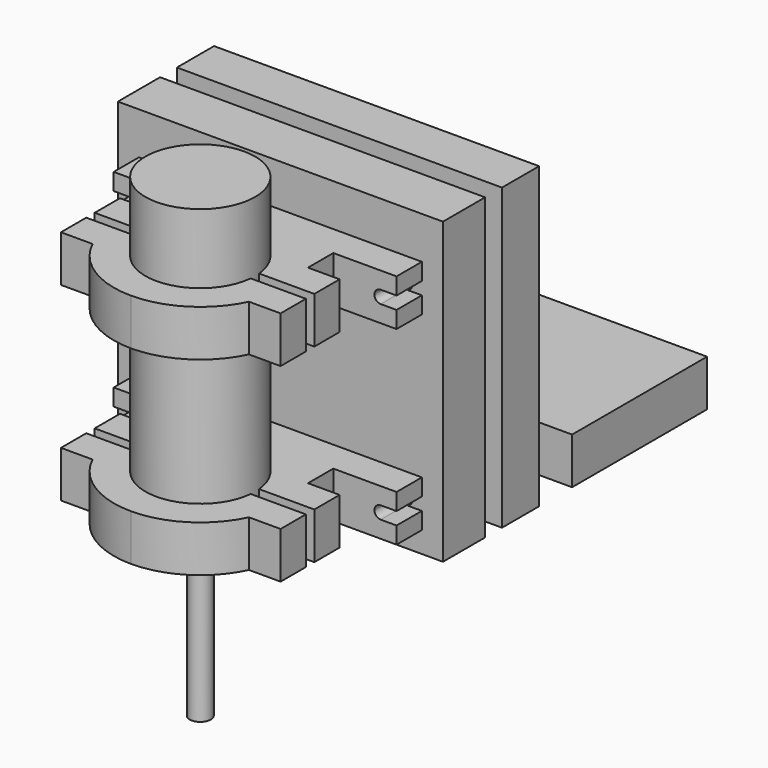
from build123d import *

# Parameters (mm, degrees)
F0_R      = 26
F0_R_2    = 5
F1_DEPTH  = 145
F2_DEPTH  = 80
F4_DEPTH  = 22
F6_DEPTH  = 88.501
F9_R      = 3
F10_DEPTH = 25
F12_W     = 154.1552425658
F12_H     = 142
F13_DEPTH = 22
F14_W     = 154.1552425658
F14_H     = 80
F15_DEPTH = 22


with BuildPart() as f1:
    # F0 (on Top) → F1 (new body)
    with BuildSketch(Plane.XY):
        Circle(F0_R)
        Circle(F0_R_2, mode=Mode.SUBTRACT)
        Circle(F0_R_2)
    extrude(amount=F1_DEPTH)

    # F0 (on Top) → F2 (join)
    with BuildSketch(Plane.XY):
        Circle(F0_R_2)
    extrude(amount=-F2_DEPTH)


with BuildPart() as f4:
    # F3 (on Top) → F4 (new body)
    with BuildSketch(Plane.XY):
        with BuildLine():
            ThreePointArc((25.8795285892, -2.5), (0, -26), (-25.8795285892, -2.5))
            Line((-25.8795285892, -2.5), (-52.0776212829, -2.5))
            Line((-52.0776212829, -2.5), (-52.0776212829, -17.5))
            Line((-52.0776212829, -17.5), (-37.0776212829, -17.5))
            ThreePointArc((-37.0776212829, -17.5), (-21.9488040676, -34.6301891418), (0, -41))
            ThreePointArc((0, -41), (21.9488040676, -34.6301891418), (37.0776212829, -17.5))
            Line((37.0776212829, -17.5), (52.0776212829, -17.5))
            Line((52.0776212829, -17.5), (52.0776212829, -2.5))
            Line((52.0776212829, -2.5), (25.8795285892, -2.5))
        make_face()
    extrude(amount=F4_DEPTH)


with BuildPart() as f4b:
    # F3 (on Top) → F4, piece 2 (new body)
    with BuildSketch(Plane.XY):
        with BuildLine():
            Line((-52.0776212829, 2.5), (-25.8795285892, 2.5))
            ThreePointArc((-25.8795285892, 2.5), (0, 26), (25.8795285892, 2.5))
            Line((25.8795285892, 2.5), (52.0776212829, 2.5))
            Line((52.0776212829, 2.5), (52.0776212829, 17.5))
            Line((52.0776212829, 17.5), (37.0776212829, 17.5))
            Line((37.0776212829, 17.5), (37.0776212829, 32.5))
            Line((37.0776212829, 32.5), (67.0776212829, 32.5))
            Line((67.0776212829, 32.5), (67.0776212829, 47.5))
            Line((67.0776212829, 47.5), (0, 47.5))
            Line((0, 47.5), (-67.0776212829, 47.5))
            Line((-67.0776212829, 47.5), (-67.0776212829, 32.5))
            Line((-67.0776212829, 32.5), (-37.0776212829, 32.5))
            Line((-37.0776212829, 32.5), (-37.0776212829, 17.5))
            Line((-37.0776212829, 17.5), (-52.0776212829, 17.5))
            Line((-52.0776212829, 17.5), (-52.0776212829, 2.5))
        make_face()
    extrude(amount=F4_DEPTH)

    # F5 (on face) → F6 (cut, through all)
    with BuildSketch(Plane(origin=(0, 47.5, 0), x_dir=(-1, 0, 0), z_dir=(0, 1, 0))):
        with BuildLine():
            ThreePointArc((-59.5776212829, 8), (-57.4563009394, 8.8786796564), (-56.5776212829, 11))
            ThreePointArc((-56.5776212829, 11), (-57.4563009394, 13.1213203436), (-59.5776212829, 14))
            ThreePointArc((-59.5776212829, 14), (-61.6989416265, 13.1213203436), (-62.5776212829, 11))
            ThreePointArc((-62.5776212829, 11), (-61.6989416265, 8.8786796564), (-59.5776212829, 8))
        make_face()
        with BuildLine():
            ThreePointArc((-62.5776212829, 11), (-61.6989416265, 13.1213203436), (-59.5776212829, 14))
            Line((-59.5776212829, 14), (-67.0776212829, 14))
            Line((-67.0776212829, 14), (-67.0776212829, 8))
            Line((-67.0776212829, 8), (-59.5776212829, 8))
            ThreePointArc((-59.5776212829, 8), (-61.6989416265, 8.8786796564), (-62.5776212829, 11))
        make_face()
        with BuildLine():
            ThreePointArc((59.5776212829, 14), (57.4563009394, 13.1213203436), (56.5776212829, 11))
            ThreePointArc((56.5776212829, 11), (57.4563009394, 8.8786796564), (59.5776212829, 8))
            ThreePointArc((59.5776212829, 8), (61.6989416265, 8.8786796564), (62.5776212829, 11))
            ThreePointArc((62.5776212829, 11), (61.6989416265, 13.1213203436), (59.5776212829, 14))
        make_face()
        with BuildLine():
            Line((67.0776212829, 14), (59.5776212829, 14))
            ThreePointArc((59.5776212829, 14), (61.6989416265, 13.1213203436), (62.5776212829, 11))
            ThreePointArc((62.5776212829, 11), (61.6989416265, 8.8786796564), (59.5776212829, 8))
            Line((59.5776212829, 8), (67.0776212829, 8))
            Line((67.0776212829, 8), (67.0776212829, 14))
        make_face()
    extrude(amount=-F6_DEPTH, mode=Mode.SUBTRACT)


with BuildPart() as f7_1:
    # F7: copy of F4
    add(f4.part.moved(Location((0, 0, 90))))


with BuildPart() as f8_1:
    # F8: copy of F4b
    add(f4b.part.moved(Location((0, 0, 90))))


with BuildPart() as f10:
    # F9 (on face) → F10 (new body)
    with BuildSketch(Plane(origin=(0, 47.5, 0), x_dir=(-1, 0, 0), z_dir=(0, 1, 0))):
        Polygon((77.0776212829, 132), (0, 132), (-77.0776212829, 132), (-77.0776212829, -10), (0, -10), (77.0776212829, -10), align=None)
        with Locations((-59.5776212829, 11)):
            Circle(F9_R, mode=Mode.SUBTRACT)
        with Locations((59.5776212829, 11)):
            Circle(F9_R, mode=Mode.SUBTRACT)
        with Locations((-59.5776212829, 101)):
            Circle(F9_R, mode=Mode.SUBTRACT)
        with Locations((59.5776212829, 101)):
            Circle(F9_R, mode=Mode.SUBTRACT)
    extrude(amount=F10_DEPTH)


with BuildPart() as f13:
    # F12 (on offset) → F13 (new body)
    with BuildSketch(Plane(origin=(0, 82.5, 0), x_dir=(-1, 0, 0), z_dir=(0, 1, 0))):
        with Locations((0, 61)):
            Rectangle(F12_W, F12_H)
    extrude(amount=F13_DEPTH)


with BuildPart() as f15:
    # F14 (on face) → F15 (new body)
    with BuildSketch(Plane(origin=(0, 0, -10), x_dir=(1, 0, 0), z_dir=(0, 0, -1))):
        with Locations((0, -164.0589302778)):
            Rectangle(F14_W, F14_H)
    extrude(amount=-F15_DEPTH)


solid = Compound([f1.part, f4.part, f4b.part, f7_1.part, f8_1.part, f10.part, f13.part, f15.part])
